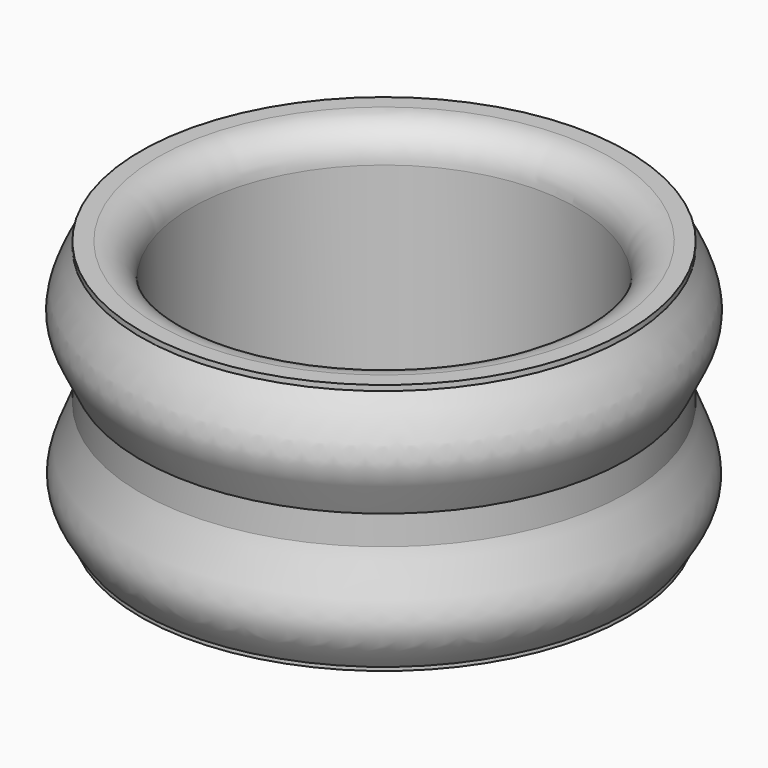
from build123d import *

# Parameters (mm, degrees)
F0_R     = 14.5
F0_R_2   = 11.5
F1_DEPTH = 15
F4_R     = 2


with BuildPart() as f1:
    # F0 (on Top) → F1 (new body)
    with BuildSketch(Plane.XY):
        Circle(F0_R)
        Circle(F0_R_2, mode=Mode.SUBTRACT)
    extrude(amount=F1_DEPTH)

    # F2 (on Right) → F3 (revolve)
    with BuildSketch(Plane.YZ):
        with BuildLine():
            Line((14.3614634871, 7.3552662202), (14.3614634871, 0))
            add(Edge.make_bspline(
                [(14.3614634871, 0), (14.9504079207, 0.9304922077), (16.6548571623, 2.8216808934), (14.4028853591, 5.9446320648), (14.3614634871, 7.3552662202)],
                knots=[0, 0, 0, 0, 0.2256215871, 0.4910996399, 0.4910996399, 0.4910996399, 0.4910996399], degree=3))
        make_face()
        with BuildLine():
            Line((14.3614634871, 14.9314038285), (14.3614634871, 7.5))
            add(Edge.make_bspline(
                [(14.3614634871, 7.5), (14.3999492825, 8.7640410433), (16.6290791491, 10.8696454885), (15.1217498865, 13.5368572633), (14.3614634871, 14.9314038285)],
                knots=[0.5002427536, 0.5002427536, 0.5002427536, 0.5002427536, 0.7415319642, 1, 1, 1, 1], degree=3))
        make_face()
    revolve(axis=Axis((0, 0, 0), (0, 0, 1)))

    # F4
    f4_edges = [f1.edges().sort_by_distance(p)[0] for p in [
        (-11.5, 0, 0),
        (-11.5, 0, 15),
    ]]
    fillet(f4_edges, radius=F4_R)


solid = f1.part
